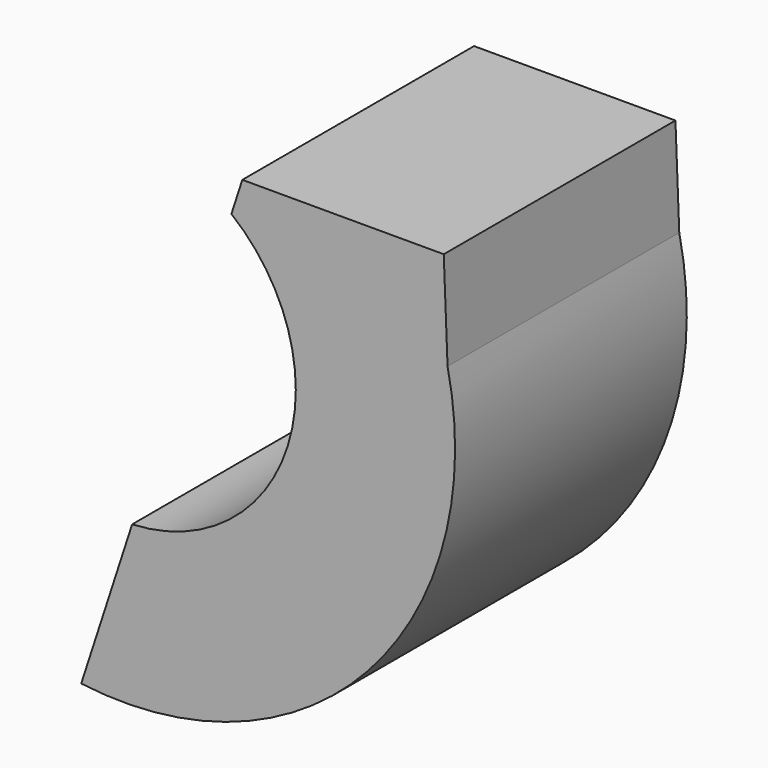
from build123d import *

# Parameters (mm, degrees)
F1_DEPTH = 7


with BuildPart() as f1:
    # F0 (on Front) → F1 (new body)
    with BuildSketch(Plane.XZ):
        with BuildLine():
            ThreePointArc((-18.6193257059, 24.4526938776), (-17.4724085616, 23.0101324022), (-17.0632034356, 21.2132034356))
            ThreePointArc((-17.0632034356, 21.2132034356), (-18.2107776829, 18.3482532441), (-21.0188369777, 17.0677575392))
            Line((-21.0188369777, 17.0677575392), (-22.249362675, 13.2805888584))
            ThreePointArc((-22.249362675, 13.2805888584), (-15.3241365798, 15.7985112404), (-13.3952950657, 22.9103506653))
            Line((-13.3952950657, 22.9103506653), (-13.4874691837, 25.2643290081))
            Line((-13.4874691837, 25.2643290081), (-18.3556094659, 25.2643290081))
            Line((-18.3556094659, 25.2643290081), (-18.6193257059, 24.4526938776))
        make_face()
    extrude(amount=F1_DEPTH)


solid = f1.part
